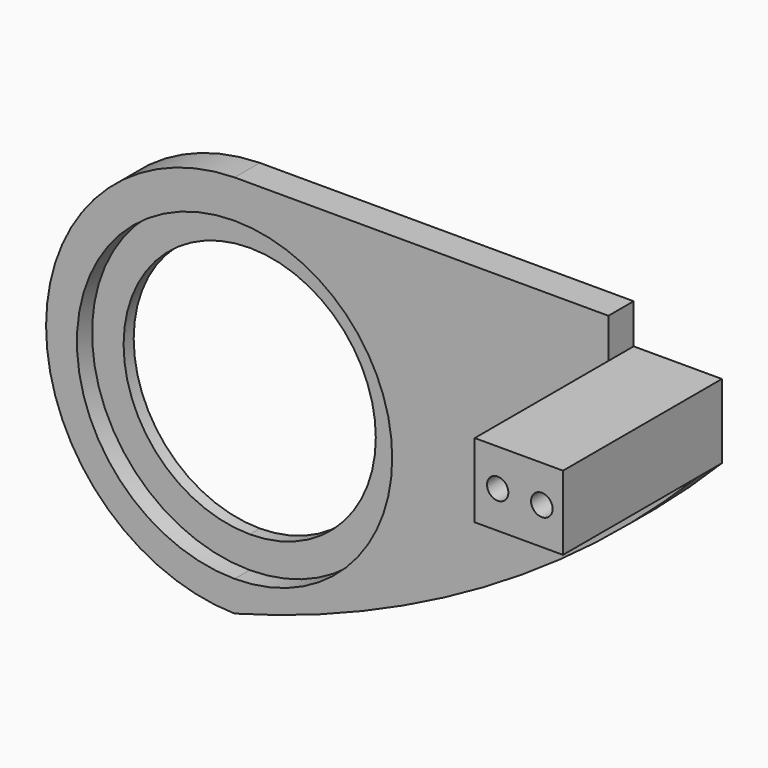
from build123d import *

# Parameters (mm, degrees)
F1_DEPTH = 5
F0_W     = 14.0000022948
F0_H     = 11.7600001395
F0_R     = 1.6916232852
F0_R_2   = 1.7089194305
F7_DEPTH = 31.5
F8_DEPTH = 2


# Not quite as in the source:
# - the program builds the solid bodies; features that only make, move or delete a surface that nothing else refers to are left out


with BuildPart() as f1:
    # F0 (on Front) → F1 (new body)
    with BuildSketch(Plane.XZ):
        with BuildLine():
            ThreePointArc((0, -25), (-25, 0), (0, 25))
            Line((0, 25), (0, 31.0474538393))
            ThreePointArc((0, 31.0474538393), (-29.8919830792, 0.5977015918), (0, -29.8520506557))
            Line((0, -29.8520506557), (0, -25))
        make_face()
        with BuildLine():
            ThreePointArc((0, 25), (17.6776695297, 17.6776695297), (25, 0))
            ThreePointArc((25, 0), (17.6776695297, -17.6776695297), (0, -25))
            Line((0, -25), (0, -29.8520506557))
            ThreePointArc((0, -29.8520506557), (39.4905936266, -13.3235446474), (73.2899941504, 12.9499975592))
            Line((73.2899941504, 12.9499975592), (59.2899918556, 12.9499975592))
            Line((59.2899918556, 12.9499975592), (59.2899918556, 24.7099976987))
            Line((59.2899918556, 24.7099976987), (59.2899918556, 31.0100000352))
            Line((59.2899918556, 31.0100000352), (0, 31.0474538393))
            Line((0, 31.0474538393), (0, 25))
        make_face()
    extrude(amount=F1_DEPTH)

    # F0 (on Front) → F7 (join)
    with BuildSketch(Plane.XZ):
        with Locations((66.289993003, 18.8299976289)):
            Rectangle(F0_W, F0_H)
        with Locations((62.9299916327, 18.8299976289)):
            Circle(F0_R, mode=Mode.SUBTRACT)
        with Locations((69.9299909174, 18.8299976289)):
            Circle(F0_R_2, mode=Mode.SUBTRACT)
    extrude(amount=F7_DEPTH)

    # F0 (on Front) → F8 (join)
    with BuildSketch(Plane.XZ):
        with BuildLine():
            ThreePointArc((0, -25), (17.6776695297, -17.6776695297), (25, 0))
            ThreePointArc((25, 0), (17.6776695297, 17.6776695297), (0, 25))
            Line((0, 25), (0, 20))
            ThreePointArc((0, 20), (14.1421356237, 14.1421356237), (20, 0))
            ThreePointArc((20, 0), (14.1421356237, -14.1421356237), (0, -20))
            Line((0, -20), (0, -25))
        make_face()
        with BuildLine():
            Line((0, 20), (0, 25))
            ThreePointArc((0, 25), (-25, 0), (0, -25))
            Line((0, -25), (0, -20))
            ThreePointArc((0, -20), (-20, 0), (0, 20))
        make_face()
    extrude(amount=F8_DEPTH)


solid = f1.part
